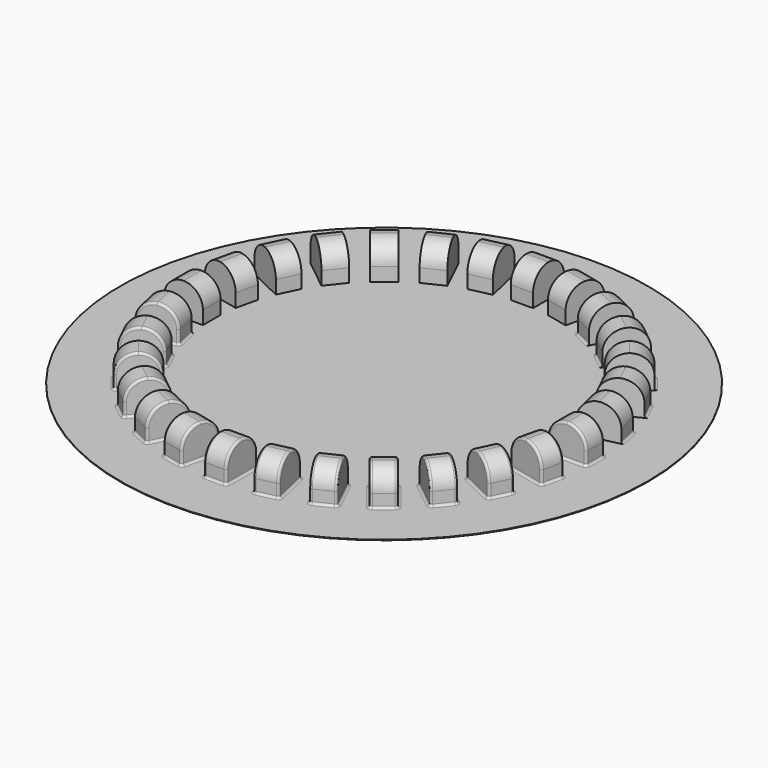
from build123d import *

# Parameters (mm, degrees)
F0_R     = 47.5
F1_DEPTH = 0.1
F2_W     = 4
F2_H     = 7
F2_W_2   = 7
F2_H_2   = 4
F3_DEPTH = 6
F4_R     = 3.49999
F5_R     = 0.4


# Not quite as in the source:
# - a fillet or chamfer is up to 0.001 mm smaller than in the source, because OpenCascade refuses the exact size


with BuildPart() as f1:
    # F0 (on Top) → F1 (new body)
    with BuildSketch(Plane.XY):
        Circle(F0_R)
    extrude(amount=F1_DEPTH)

    # F2 (on Top) → F3 (join)
    with BuildSketch(Plane.XY):
        with Locations((0, 34.5)):
            Rectangle(F2_W, F2_H)
        Polygon((-10.4056513147, 36.602218795), (-8.848004777, 29.7777234097), (-4.9482931283, 30.6678071455), (-6.505939666, 37.4923025308), align=None)
        Polygon((-18.2895198223, 33.3690495021), (-15.2523336484, 27.0622674267), (-11.6484581768, 28.7978023832), (-14.6856443507, 35.1045844585), align=None)
        Polygon((-25.2562754356, 28.4626167301), (-20.8918468226, 22.9897963528), (-17.7645208927, 25.4837555602), (-22.1289495057, 30.9565759375), align=None)
        Polygon((-30.9565759375, 22.1289495057), (-25.4837555602, 17.7645208927), (-22.9897963528, 20.8918468226), (-28.4626167301, 25.2562754356), align=None)
        Polygon((-35.1045844585, 14.6856443507), (-28.7978023832, 11.6484581768), (-27.0622674267, 15.2523336484), (-33.3690495021, 18.2895198223), align=None)
        Polygon((-37.4923025308, 6.505939666), (-30.6678071455, 4.9482931283), (-29.7777234097, 8.848004777), (-36.602218795, 10.4056513147), align=None)
        with Locations((-34.5, 0)):
            Rectangle(F2_W_2, F2_H_2)
        Polygon((-36.602218795, -10.4056513147), (-29.7777234097, -8.848004777), (-30.6678071455, -4.9482931283), (-37.4923025308, -6.505939666), align=None)
        Polygon((-33.3690495021, -18.2895198223), (-27.0622674267, -15.2523336484), (-28.7978023832, -11.6484581768), (-35.1045844585, -14.6856443507), align=None)
        Polygon((-28.4626167301, -25.2562754356), (-22.9897963528, -20.8918468226), (-25.4837555602, -17.7645208927), (-30.9565759375, -22.1289495057), align=None)
        Polygon((-22.1289495057, -30.9565759375), (-17.7645208927, -25.4837555602), (-20.8918468226, -22.9897963528), (-25.2562754356, -28.4626167301), align=None)
        Polygon((-14.6856443507, -35.1045844585), (-11.6484581768, -28.7978023832), (-15.2523336484, -27.0622674267), (-18.2895198223, -33.3690495021), align=None)
        Polygon((-6.505939666, -37.4923025308), (-4.9482931283, -30.6678071455), (-8.848004777, -29.7777234097), (-10.4056513147, -36.602218795), align=None)
        with Locations((0, -34.5)):
            Rectangle(F2_W, F2_H)
        Polygon((10.4056513147, -36.602218795), (8.848004777, -29.7777234097), (4.9482931283, -30.6678071455), (6.505939666, -37.4923025308), align=None)
        Polygon((18.2895198223, -33.3690495021), (15.2523336484, -27.0622674267), (11.6484581768, -28.7978023832), (14.6856443507, -35.1045844585), align=None)
        Polygon((25.2562754356, -28.4626167301), (20.8918468226, -22.9897963528), (17.7645208927, -25.4837555602), (22.1289495057, -30.9565759375), align=None)
        Polygon((30.9565759375, -22.1289495057), (25.4837555602, -17.7645208927), (22.9897963528, -20.8918468226), (28.4626167301, -25.2562754356), align=None)
        Polygon((35.1045844585, -14.6856443507), (28.7978023832, -11.6484581768), (27.0622674267, -15.2523336484), (33.3690495021, -18.2895198223), align=None)
        Polygon((37.4923025308, -6.505939666), (30.6678071455, -4.9482931283), (29.7777234097, -8.848004777), (36.602218795, -10.4056513147), align=None)
        with Locations((34.5, 0)):
            Rectangle(F2_W_2, F2_H_2)
        Polygon((36.602218795, 10.4056513147), (29.7777234097, 8.848004777), (30.6678071455, 4.9482931283), (37.4923025308, 6.505939666), align=None)
        Polygon((33.3690495021, 18.2895198223), (27.0622674267, 15.2523336484), (28.7978023832, 11.6484581768), (35.1045844585, 14.6856443507), align=None)
        Polygon((28.4626167301, 25.2562754356), (22.9897963528, 20.8918468226), (25.4837555602, 17.7645208927), (30.9565759375, 22.1289495057), align=None)
        Polygon((22.1289495057, 30.9565759375), (17.7645208927, 25.4837555602), (20.8918468226, 22.9897963528), (25.2562754356, 28.4626167301), align=None)
        Polygon((14.6856443507, 35.1045844585), (11.6484581768, 28.7978023832), (15.2523336484, 27.0622674267), (18.2895198223, 33.3690495021), align=None)
        Polygon((6.505939666, 37.4923025308), (4.9482931283, 30.6678071455), (8.848004777, 29.7777234097), (10.4056513147, 36.602218795), align=None)
    extrude(amount=F3_DEPTH)

    # F4 (radius 3.5 in the source; OpenCascade refuses exactly that, so slightly less here)
    f4_edges = [f1.edges().sort_by_distance(p)[0] for p in [
        (-6.898149, 30.222765, 6),
        (0, 31, 6),
        (6.898149, 30.222765, 6),
        (13.450396, 27.930035, 6),
        (19.328184, 24.236776, 6),
        (24.236776, 19.328184, 6),
        (27.930035, 13.450396, 6),
        (30.222765, 6.898149, 6),
        (31, 0, 6),
        (30.222765, -6.898149, 6),
        (27.930035, -13.450396, 6),
        (24.236776, -19.328184, 6),
        (19.328184, -24.236776, 6),
        (13.450396, -27.930035, 6),
        (6.898149, -30.222765, 6),
        (0, -31, 6),
        (-6.898149, -30.222765, 6),
        (-13.450396, -27.930035, 6),
        (-19.328184, -24.236776, 6),
        (-24.236776, -19.328184, 6),
        (-27.930035, -13.450396, 6),
        (-30.222765, -6.898149, 6),
        (-31, 0, 6),
        (-30.222765, 6.898149, 6),
        (-27.930035, 13.450396, 6),
        (-24.236776, 19.328184, 6),
        (-19.328184, 24.236776, 6),
        (-13.450396, 27.930035, 6),
        (-8.455795, 37.047261, 6),
        (0, 38, 6),
        (8.455795, 37.047261, 6),
        (16.487582, 34.236817, 6),
        (23.692612, 29.709596, 6),
        (29.709596, 23.692612, 6),
        (34.236817, 16.487582, 6),
        (37.047261, 8.455795, 6),
        (38, 0, 6),
        (37.047261, -8.455795, 6),
        (34.236817, -16.487582, 6),
        (29.709596, -23.692612, 6),
        (23.692612, -29.709596, 6),
        (16.487582, -34.236817, 6),
        (8.455795, -37.047261, 6),
        (0, -38, 6),
        (-8.455795, -37.047261, 6),
        (-16.487582, -34.236817, 6),
        (-23.692612, -29.709596, 6),
        (-29.709596, -23.692612, 6),
        (-34.236817, -16.487582, 6),
        (-37.047261, -8.455795, 6),
        (-38, 0, 6),
        (-37.047261, 8.455795, 6),
        (-34.236817, 16.487582, 6),
        (-29.709596, 23.692612, 6),
        (-23.692612, 29.709596, 6),
        (-16.487582, 34.236817, 6),
    ]]
    fillet(f4_edges, radius=F4_R)

    # F5
    f5_edges = [f1.edges().sort_by_distance(p)[0] for p in [
        (11.648458, 28.797802, 1.300005),
        (12.093243, 29.721407, 4.974877),
        (13.167051, 31.951193, 0.1),
        (13.167051, 31.951193, 6),
        (14.685644, 35.104584, 1.300005),
        (14.24086, 34.18098, 4.974877),
        (17.764521, 25.483756, 1.300005),
        (18.403675, 26.285229, 4.974877),
        (19.946735, 28.220166, 0.1),
        (19.946735, 28.220166, 6),
        (22.12895, 30.956576, 1.300005),
        (21.489796, 30.155102, 4.974877),
        (22.989796, 20.891847, 1.300005),
        (23.79127, 21.531001, 4.974877),
        (25.726207, 23.074061, 0.1),
        (25.726207, 23.074061, 6),
        (28.462617, 25.256275, 1.300005),
        (27.661143, 24.617121, 4.974877),
        (27.062267, 15.252334, 1.300005),
        (27.985872, 15.697118, 4.974877),
        (30.215658, 16.770927, 0.1),
        (30.215658, 16.770927, 6),
        (33.36905, 18.28952, 1.300005),
        (32.445445, 17.844735, 4.974877),
        (29.777723, 8.848005, 1.300005),
        (30.777145, 9.076116, 4.974877),
        (33.189971, 9.626828, 0.1),
        (33.189971, 9.626828, 6),
        (36.602219, 10.405651, 1.300005),
        (35.602797, 10.17754, 4.974877),
        (31, 2, 1.300005),
        (32.025123, 2, 4.974877),
        (34.5, 2, 0.1),
        (34.5, 2, 6),
        (38, 2, 1.300005),
        (36.974877, 2, 4.974877),
        (30.667807, -4.948293, 1.300005),
        (31.667229, -5.176405, 4.974877),
        (34.080055, -5.727116, 0.1),
        (34.080055, -5.727116, 6),
        (37.492303, -6.50594, 1.300005),
        (36.492881, -6.277828, 4.974877),
        (28.797802, -11.648458, 1.300005),
        (29.721407, -12.093243, 4.974877),
        (31.951193, -13.167051, 0.1),
        (31.951193, -13.167051, 6),
        (35.104584, -14.685644, 1.300005),
        (34.18098, -14.24086, 4.974877),
        (25.483756, -17.764521, 1.300005),
        (26.285229, -18.403675, 4.974877),
        (28.220166, -19.946735, 0.1),
        (28.220166, -19.946735, 6),
        (30.956576, -22.12895, 1.300005),
        (30.155102, -21.489796, 4.974877),
        (20.891847, -22.989796, 1.300005),
        (21.531001, -23.79127, 4.974877),
        (23.074061, -25.726207, 0.1),
        (23.074061, -25.726207, 6),
        (25.256275, -28.462617, 1.300005),
        (24.617121, -27.661143, 4.974877),
        (15.252334, -27.062267, 1.300005),
        (15.697118, -27.985872, 4.974877),
        (16.770927, -30.215658, 0.1),
        (16.770927, -30.215658, 6),
        (18.28952, -33.36905, 1.300005),
        (17.844735, -32.445445, 4.974877),
        (33.36905, -18.28952, 1.300005),
        (32.445445, -17.844735, 4.974877),
        (30.215658, -16.770927, 0.1),
        (30.215658, -16.770927, 6),
        (27.062267, -15.252334, 1.300005),
        (27.985872, -15.697118, 4.974877),
        (36.602219, -10.405651, 1.300005),
        (35.602797, -10.17754, 4.974877),
        (33.189971, -9.626828, 0.1),
        (33.189971, -9.626828, 6),
        (29.777723, -8.848005, 1.300005),
        (30.777145, -9.076116, 4.974877),
        (38, -2, 1.300005),
        (36.974877, -2, 4.974877),
        (34.5, -2, 0.1),
        (34.5, -2, 6),
        (31, -2, 1.300005),
        (32.025123, -2, 4.974877),
        (28.462617, -25.256275, 1.300005),
        (27.661143, -24.617121, 4.974877),
        (25.726207, -23.074061, 0.1),
        (25.726207, -23.074061, 6),
        (22.989796, -20.891847, 1.300005),
        (23.79127, -21.531001, 4.974877),
        (22.12895, -30.956576, 1.300005),
        (21.489796, -30.155102, 4.974877),
        (19.946735, -28.220166, 0.1),
        (19.946735, -28.220166, 6),
        (17.764521, -25.483756, 1.300005),
        (18.403675, -26.285229, 4.974877),
        (14.685644, -35.104584, 1.300005),
        (14.24086, -34.18098, 4.974877),
        (13.167051, -31.951193, 0.1),
        (13.167051, -31.951193, 6),
        (11.648458, -28.797802, 1.300005),
        (12.093243, -29.721407, 4.974877),
        (8.848005, -29.777723, 1.300005),
        (9.076116, -30.777145, 4.974877),
        (9.626828, -33.189971, 0.1),
        (9.626828, -33.189971, 6),
        (10.405651, -36.602219, 1.300005),
        (10.17754, -35.602797, 4.974877),
        (6.50594, -37.492303, 1.300005),
        (6.277828, -36.492881, 4.974877),
        (5.727116, -34.080055, 0.1),
        (5.727116, -34.080055, 6),
        (4.948293, -30.667807, 1.300005),
        (5.176405, -31.667229, 4.974877),
        (2, -31, 1.300005),
        (2, -32.025123, 4.974877),
        (2, -34.5, 0.1),
        (2, -34.5, 6),
        (2, -38, 1.300005),
        (2, -36.974877, 4.974877),
        (-2, -38, 1.300005),
        (-2, -36.974877, 4.974877),
        (-2, -34.5, 0.1),
        (-2, -34.5, 6),
        (-2, -31, 1.300005),
        (-2, -32.025123, 4.974877),
        (-4.948293, -30.667807, 1.300005),
        (-5.176405, -31.667229, 4.974877),
        (-5.727116, -34.080055, 0.1),
        (-5.727116, -34.080055, 6),
        (-6.50594, -37.492303, 1.300005),
        (-6.277828, -36.492881, 4.974877),
        (-10.405651, -36.602219, 1.300005),
        (-10.17754, -35.602797, 4.974877),
        (-9.626828, -33.189971, 0.1),
        (-9.626828, -33.189971, 6),
        (-8.848005, -29.777723, 1.300005),
        (-9.076116, -30.777145, 4.974877),
        (-11.648458, -28.797802, 1.300005),
        (-12.093243, -29.721407, 4.974877),
        (-13.167051, -31.951193, 0.1),
        (-13.167051, -31.951193, 6),
        (-14.685644, -35.104584, 1.300005),
        (-14.24086, -34.18098, 4.974877),
        (-18.28952, -33.36905, 1.300005),
        (-17.844735, -32.445445, 4.974877),
        (-16.770927, -30.215658, 0.1),
        (-16.770927, -30.215658, 6),
        (-15.252334, -27.062267, 1.300005),
        (-15.697118, -27.985872, 4.974877),
        (-17.764521, -25.483756, 1.300005),
        (-18.403675, -26.285229, 4.974877),
        (-19.946735, -28.220166, 0.1),
        (-19.946735, -28.220166, 6),
        (-22.12895, -30.956576, 1.300005),
        (-21.489796, -30.155102, 4.974877),
        (-25.256275, -28.462617, 1.300005),
        (-24.617121, -27.661143, 4.974877),
        (-23.074061, -25.726207, 0.1),
        (-23.074061, -25.726207, 6),
        (-20.891847, -22.989796, 1.300005),
        (-21.531001, -23.79127, 4.974877),
        (-22.989796, -20.891847, 1.300005),
        (-23.79127, -21.531001, 4.974877),
        (-25.726207, -23.074061, 0.1),
        (-25.726207, -23.074061, 6),
        (-28.462617, -25.256275, 1.300005),
        (-27.661143, -24.617121, 4.974877),
        (-30.956576, -22.12895, 1.300005),
        (-30.155102, -21.489796, 4.974877),
        (-28.220166, -19.946735, 0.1),
        (-28.220166, -19.946735, 6),
        (-25.483756, -17.764521, 1.300005),
        (-26.285229, -18.403675, 4.974877),
        (-27.062267, -15.252334, 1.300005),
        (-27.985872, -15.697118, 4.974877),
        (-30.215658, -16.770927, 0.1),
        (-30.215658, -16.770927, 6),
        (-33.36905, -18.28952, 1.300005),
        (-32.445445, -17.844735, 4.974877),
        (-35.104584, -14.685644, 1.300005),
        (-34.18098, -14.24086, 4.974877),
        (-31.951193, -13.167051, 0.1),
        (-31.951193, -13.167051, 6),
        (-28.797802, -11.648458, 1.300005),
        (-29.721407, -12.093243, 4.974877),
        (-29.777723, -8.848005, 1.300005),
        (-30.777145, -9.076116, 4.974877),
        (-33.189971, -9.626828, 0.1),
        (-33.189971, -9.626828, 6),
        (-36.602219, -10.405651, 1.300005),
        (-35.602797, -10.17754, 4.974877),
        (-19.328184, -24.236776, 0.1),
        (-23.692612, -29.709596, 0.1),
        (-29.709596, -23.692612, 0.1),
        (-24.236776, -19.328184, 0.1),
        (-16.487582, -34.236817, 0.1),
        (-13.450396, -27.930035, 0.1),
        (-6.898149, -30.222765, 0.1),
        (-8.455795, -37.047261, 0.1),
        (-27.930035, -13.450396, 0.1),
        (-34.236817, -16.487582, 0.1),
        (-30.222765, -6.898149, 0.1),
        (-37.047261, -8.455795, 0.1),
        (0, -31, 0.1),
        (0, -38, 0.1),
        (6.898149, -30.222765, 0.1),
        (8.455795, -37.047261, 0.1),
        (13.450396, -27.930035, 0.1),
        (16.487582, -34.236817, 0.1),
        (19.328184, -24.236776, 0.1),
        (23.692612, -29.709596, 0.1),
        (29.709596, -23.692612, 0.1),
        (24.236776, -19.328184, 0.1),
        (34.236817, -16.487582, 0.1),
        (27.930035, -13.450396, 0.1),
        (30.222765, -6.898149, 0.1),
        (37.047261, -8.455795, 0.1),
        (31, 0, 0.1),
        (38, 0, 0.1),
        (30.222765, 6.898149, 0.1),
        (37.047261, 8.455795, 0.1),
        (27.930035, 13.450396, 0.1),
        (34.236817, 16.487582, 0.1),
        (16.487582, 34.236817, 0.1),
        (13.450396, 27.930035, 0.1),
        (24.236776, 19.328184, 0.1),
        (29.709596, 23.692612, 0.1),
        (19.328184, 24.236776, 0.1),
        (23.692612, 29.709596, 0.1),
    ]]
    fillet(f5_edges, radius=F5_R)


solid = f1.part
